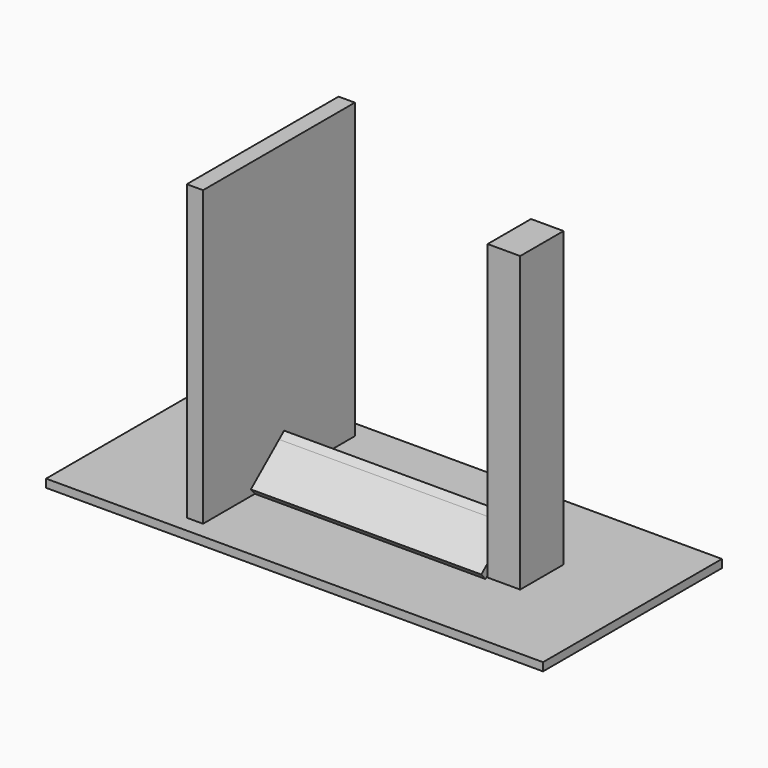
from build123d import *

# Parameters (mm, degrees)
F0_W     = 1100
F0_H     = 495
F1_DEPTH = 18
F2_W     = 36
F2_H     = 420
F3_DEPTH = 650
F2_W_2   = 72
F2_H_2   = 120
F4_W     = 120
F4_H     = 650
F5_DEPTH = 899.4299889932
F7_DEPTH = 650
F9_DEPTH = 510


# Not quite as in the source:
# - a feature names something its author has since deleted; it is built from what else it names


with BuildPart() as f1:
    # F0 (on Top) → F1 (new body)
    with BuildSketch(Plane.XY):
        Rectangle(F0_W, F0_H)
    extrude(amount=F1_DEPTH)


with BuildPart() as f3:
    # F2 (on face) → F3 (new body)
    with BuildSketch(Plane.XY.offset(18)):
        with Locations((-250.5710110068, 0)):
            Rectangle(F2_W, F2_H)
    extrude(amount=F3_DEPTH)


with BuildPart() as f3b:
    # F2 (on face) → F3, piece 2 (new body)
    with BuildSketch(Plane.XY.offset(18)):
        with Locations((313.4289889932, 0)):
            Rectangle(F2_W_2, F2_H_2)
    extrude(amount=F3_DEPTH)


with BuildPart() as f5_tool:
    # F4 (on face) → F5 (new body, through all)
    with BuildSketch(Plane.YZ.offset(349.4289889932)):
        with Locations((0, 343)):
            Rectangle(F4_W, F4_H)
    extrude(amount=-F5_DEPTH)


with BuildPart() as f3_1:
    add(f3.part)

    # F5: cut by f5_tool
    add(f5_tool.part, mode=Mode.SUBTRACT)

    # F2 (on face) → F7 (join)
    with BuildSketch(Plane.XY.offset(18)):
        with Locations((-250.5710110068, 0)):
            Rectangle(F2_W, F2_H)
    extrude(amount=F7_DEPTH)


with BuildPart() as f3b_1:
    add(f3b.part)

    # F5: cut by f5_tool
    add(f5_tool.part, mode=Mode.SUBTRACT)


with BuildPart() as f7:
    # F2 (on face) → F7, piece 2 (new body)
    with BuildSketch(Plane.XY.offset(18)):
        with Locations((313.4289889932, 0)):
            Rectangle(F2_W_2, F2_H_2)
    extrude(amount=F7_DEPTH)


with BuildPart() as f9:
    # F8 (on face) → F9 (new body)
    with BuildSketch(Plane(origin=(277.4289889932, 0, 0), x_dir=(0, -1, 0), z_dir=(-1, 0, 0))):
        Polygon((-0.5010100179, 96.7448346812), (-14.289809994, 108.3150116555), (-60, 53.8397284977), (-60, 25.8366996142), (-12.0711869922, 82.956034705), align=None)
        Polygon((60, 45.9784594893), (-0.5010100179, 96.7448346812), (-12.0711869922, 82.956034705), (60, 22.4811282813), align=None)
        Polygon((77.6355231803, 31.1804984931), (60, 45.9784594893), (60, 22.4811282813), (66.0653462059, 17.391698517), align=None)
        Polygon((-60, 25.8366996142), (-60, 53.8397284977), (-79.854146182, 30.1784784574), (-66.0653462059, 18.608301483), align=None)
    extrude(amount=F9_DEPTH)


solid = Compound([f1.part, f3_1.part, f7.part, f9.part])
